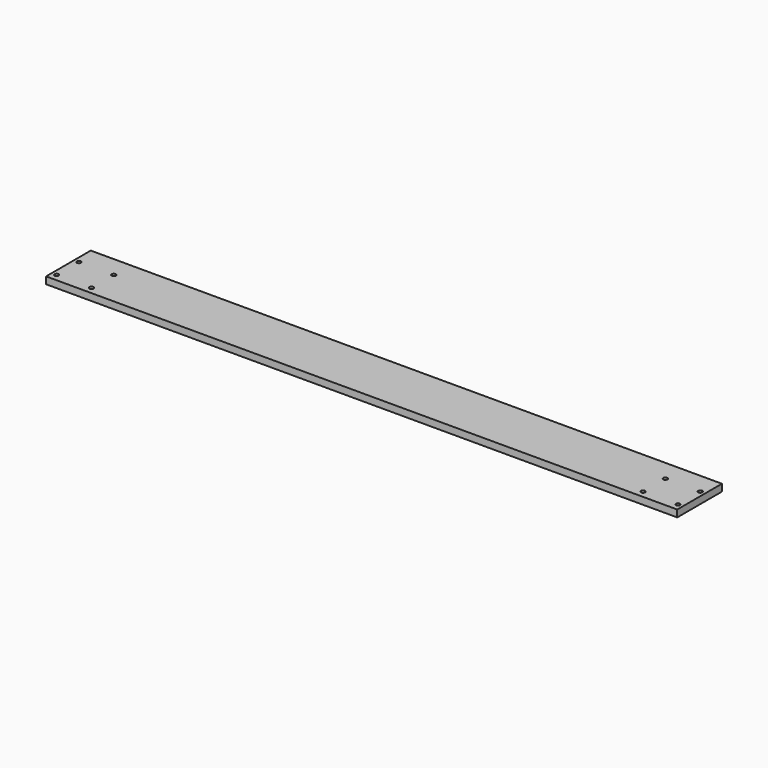
from build123d import *

# Parameters (mm, degrees)
F0_W     = 452
F0_H     = 40
F0_W_2   = 25
F0_H_2   = 20
F1_DEPTH = 5
F2_D     = 3


# Not quite as in the source:
# - a feature names something its author has since deleted; it is built from what else it names


with BuildPart() as f1:
    # F0 (on Top) → F1 (new body)
    with BuildSketch(Plane.XY):
        with Locations((0, 15)):
            Rectangle(F0_W, F0_H)
        with Locations((-210, 10)):
            Rectangle(F0_W_2, F0_H_2, mode=Mode.SUBTRACT)
        with Locations((210, 10)):
            Rectangle(F0_W_2, F0_H_2, mode=Mode.SUBTRACT)
        with Locations((210, 10)):
            Rectangle(F0_W_2, F0_H_2)
        with Locations((-210, 10)):
            Rectangle(F0_W_2, F0_H_2)
    extrude(amount=F1_DEPTH)

    # F2 (through all)
    with Locations(Plane(origin=(0, 0, 0), x_dir=(1, 0, 0), z_dir=(0, 0, -1))):
        with Locations((-222.5, 0), (-197.5, 0), (197.5, 0), (222.5, 0), (-222.5, -20), (-197.5, -20), (222.5, -20), (197.5, -20)):
            Hole(F2_D / 2)


solid = f1.part
